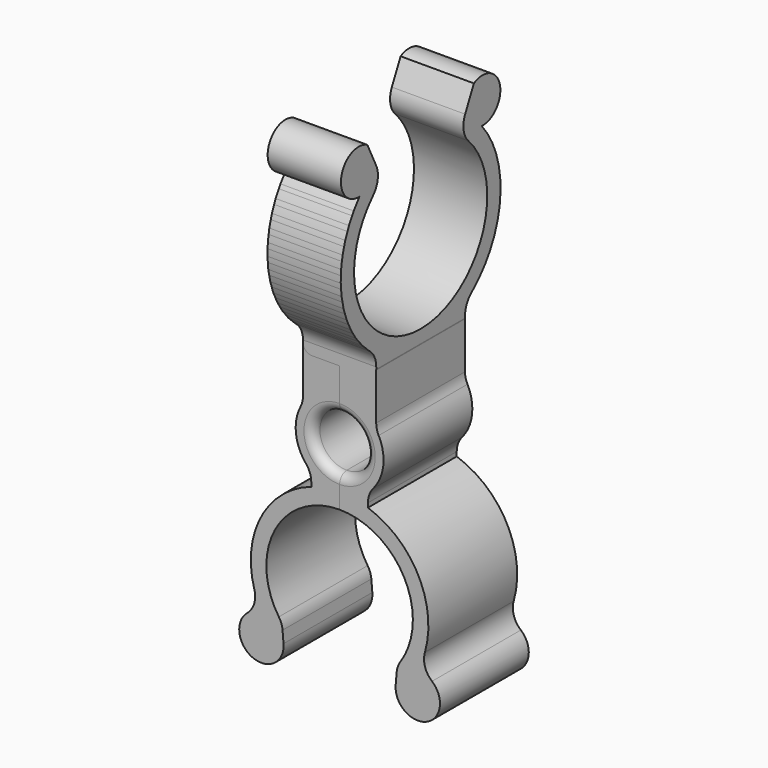
from build123d import *

# Parameters (mm, degrees)
F1_DEPTH = 25
F3_DEPTH = 16.5
F5_R     = 5
F5_2_R   = 5
F6_R     = 2
F6_2_R   = 2


with BuildPart() as f1:
    # F0 (on Front) → F1 (new body)
    with BuildSketch(Plane.XZ):
        with BuildLine():
            ThreePointArc((0, -13.0244963626), (14.841258851, -22.3142927791), (12.9707270003, -39.7230374879))
            Line((12.9707270003, -39.7230374879), (12.6301857194, -43.7085150799))
            ThreePointArc((12.6301857194, -43.7085150799), (21.0202444261, -47.7926193342), (17.539775381, -39.1347138203))
            ThreePointArc((17.539775381, -39.1347138203), (18.6284646808, -22.2457393509), (6.3781159631, -10.5687680263))
            Line((6.3781159631, -10.5687680263), (6.3781159631, -7.5687680263))
            ThreePointArc((6.3781159631, -7.5687680263), (9.7979360751, -1.4025196408), (8.2453303507, 5.4755036374))
            Line((8.2453303507, 5.4755036374), (8.2453303507, 15.4755036374))
            Line((8.2453303507, 15.4755036374), (0, 15.4755036374))
            Line((0, 15.4755036374), (0, 6.0244963626))
            ThreePointArc((0, 6.0244963626), (6.0244963626, 0), (0, -6.0244963626))
            Line((0, -6.0244963626), (0, -13.0244963626))
        make_face()
    extrude(amount=F1_DEPTH)

    # F2 (on face) → F3 (join)
    with BuildSketch(Plane.YZ.offset(8.2453303507)):
        with BuildLine():
            ThreePointArc((-1.6496046584, 54.4491597502), (-12.5, 20.4076123815), (-23.3503953416, 54.4491597502))
            Line((-23.3503953416, 54.4491597502), (-25.001859694, 57.8541294423))
            Line((-25.001859694, 57.8541294423), (-25.0057154727, 57.8620792414))
            Line((-25.0057154727, 57.8620792414), (-27.5, 63.0047656136))
            ThreePointArc((-27.5, 63.0047656136), (-34.8052642949, 59.7918207884), (-29.7149281613, 53.6454089151))
            ThreePointArc((-29.7149281613, 53.6454089151), (-34.7764276378, 35.993632025), (-25, 20.4493254476))
            Line((-25, 20.4493254476), (-25, 15.4755036374))
            Line((-25, 15.4755036374), (0, 15.4755036374))
            Line((0, 15.4755036374), (0, 20.4493254476))
            ThreePointArc((0, 20.4493254476), (9.7764276378, 35.993632025), (4.7149281613, 53.6454089151))
            ThreePointArc((4.7149281613, 53.6454089151), (9.8052642949, 59.7918207884), (2.5, 63.0047656136))
            Line((2.5, 63.0047656136), (0.0057154727, 57.8620792414))
            Line((0.0057154727, 57.8620792414), (0.001859694, 57.8541294423))
            Line((0.001859694, 57.8541294423), (-1.6496046584, 54.4491597502))
        make_face()
    extrude(amount=-F3_DEPTH)


with BuildPart() as f4_1:
    # F4: instance of F1
    add(f1.part.mirror(Plane.YZ))

    # F5#2
    f5_2_edges = [f4_1.edges().sort_by_distance(p)[0] for p in [
        (-12.970727, -12.5, -39.723037),
        (-17.539775, -12.5, -39.134714),
        (-8.24533, -12.5, 5.475504),
        (-6.378116, -12.5, -7.568768),
        (0.00467, 0, 20.449325),
        (0.00467, -25, 20.449325),
        (0.00467, -1.649605, 54.44916),
        (0.00467, -23.350395, 54.44916),
    ]]
    fillet(f5_2_edges, radius=F5_2_R)

    # F6#2
    f6_2_edges = [f4_1.edges().sort_by_distance(p)[0] for p in [
        (-6.024496, -25, 0),
        (-6.024496, 0, 0),
        (8.25467, -12.5, 15.475504),
    ]]
    fillet(f6_2_edges, radius=F6_2_R)


with BuildPart() as f1_1:
    add(f1.part)

    # F5
    f5_edges = [f1_1.edges().sort_by_distance(p)[0] for p in [
        (12.970727, -12.5, -39.723037),
        (17.539775, -12.5, -39.134714),
        (8.24533, -12.5, 5.475504),
        (6.378116, -12.5, -7.568768),
        (-0.00467, -1.649605, 54.44916),
        (-0.00467, -23.350395, 54.44916),
    ]]
    fillet(f5_edges, radius=F5_R)

    # F6
    f6_edges = [f1_1.edges().sort_by_distance(p)[0] for p in [
        (6.024496, -25, 0),
        (6.024496, 0, 0),
        (-8.25467, -12.5, 15.475504),
    ]]
    fillet(f6_edges, radius=F6_R)


solid = Compound([f4_1.part, f1_1.part])
